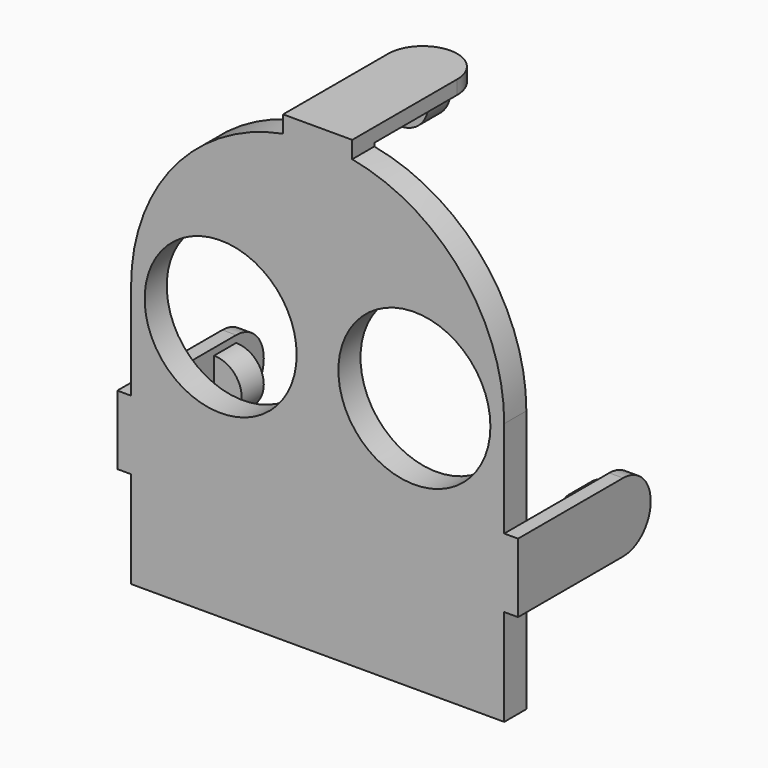
from build123d import *

# Parameters (mm, degrees)
F1_DEPTH  = 2
F4_DEPTH  = 1
F6_DEPTH  = 2
F9_DEPTH  = 1
F12_DEPTH = 1
F13_W     = 2
F13_H     = 2
F14_ANGLE = 180
F15_W     = 2
F15_H     = 2
F16_ANGLE = 180
F17_W     = 2
F17_H     = 2
F18_ANGLE = 180
F19_R     = 5.5
F20_DEPTH = 5


# Not quite as in the source:
# - a feature names something its author has since deleted; it is built from what else it names


with BuildPart() as f1:
    # F0 (on Front) → F1 (new body)
    with BuildSketch(Plane.XZ):
        with BuildLine():
            ThreePointArc((-13.5, 0), (0, -13.5), (13.5, 0))
            ThreePointArc((13.5, 0), (0, 13.5), (-13.5, 0))
        make_face()
        with BuildLine():
            Line((13.5, -19), (13.5, 0))
            ThreePointArc((13.5, 0), (0, -13.5), (-13.5, 0))
            Line((-13.5, 0), (-13.5, -19))
            Line((-13.5, -19), (13.5, -19))
        make_face()
    extrude(amount=F1_DEPTH)

    # F3 (on offset) → F4 (join)
    with BuildSketch(Plane.XY.offset(13.5)):
        with BuildLine():
            Line((-2.5, 7.5), (-2.5, -2))
            Line((-2.5, -2), (2.5, -2))
            Line((2.5, -2), (2.5, 7.5))
            ThreePointArc((2.5, 7.5), (1.767766953, 9.267766953), (0, 10))
            ThreePointArc((0, 10), (-1.767766953, 9.267766953), (-2.5, 7.5))
        make_face()
    extrude(amount=F4_DEPTH)

    # F5 (on face) → F6 (join)
    with BuildSketch(Plane.XZ.offset(2)):
        with BuildLine():
            Line((-2.5, 13.5), (-2.5, 13.2664991614))
            ThreePointArc((-2.5, 13.2664991614), (-1.2554404249, 13.4414980318), (0, 13.5))
            Line((0, 13.5), (-2.5, 13.5))
        make_face()
        with BuildLine():
            ThreePointArc((0, 13.5), (1.2554404249, 13.4414980318), (2.5, 13.2664991614))
            Line((2.5, 13.2664991614), (2.5, 13.5))
            Line((2.5, 13.5), (0, 13.5))
        make_face()
    extrude(amount=-F6_DEPTH)

    # F8 (on offset) → F9 (join)
    with BuildSketch(Plane.YZ.offset(13.5)):
        with BuildLine():
            Line((7.5, -7), (-2, -7))
            Line((-2, -7), (-2, -12))
            Line((-2, -12), (7.5, -12))
            ThreePointArc((7.5, -12), (9.267766953, -11.267766953), (10, -9.5))
            ThreePointArc((10, -9.5), (9.267766953, -7.732233047), (7.5, -7))
        make_face()
    extrude(amount=F9_DEPTH)

    # F11 (on offset) → F12 (join)
    with BuildSketch(Plane.YZ.offset(-13.5)):
        with BuildLine():
            Line((7.5, -7), (-2, -7))
            Line((-2, -7), (-2, -12))
            Line((-2, -12), (7.5, -12))
            ThreePointArc((7.5, -12), (9.267766953, -11.267766953), (10, -9.5))
            ThreePointArc((10, -9.5), (9.267766953, -7.732233047), (7.5, -7))
        make_face()
    extrude(amount=-F12_DEPTH)

    # F13 (on face) → F14 (revolve)
    with BuildSketch(Plane(origin=(0, 0, 13.5), x_dir=(1, 0, 0), z_dir=(0, 0, -1))):
        with Locations((-1, -6.5)):
            Rectangle(F13_W, F13_H)
    revolve(axis=Axis((0, 6.5, 13.5), (0, -1, 0)), revolution_arc=F14_ANGLE)

    # F15 (on face) → F16 (revolve)
    with BuildSketch(Plane(origin=(13.5, 0, 0), x_dir=(0, -1, 0), z_dir=(-1, 0, 0))):
        with Locations((-6.5, -8.5)):
            Rectangle(F15_W, F15_H)
    revolve(axis=Axis((13.5, 6.5, -9.5), (0, -1, 0)), revolution_arc=F16_ANGLE)

    # F17 (on face) → F18 (revolve)
    with BuildSketch(Plane.YZ.offset(-13.5)):
        with Locations((6.5, -8.5)):
            Rectangle(F17_W, F17_H)
    revolve(axis=Axis((-13.5, 6.5, -9.5), (0, 1, 0)), revolution_arc=F18_ANGLE)

    # F19 (on face) → F20 (cut)
    with BuildSketch(Plane.XZ.offset(2)):
        with Locations((-7.0192593016, -0.5)):
            Circle(F19_R)
        with Locations((7, -0.5)):
            Circle(F19_R)
    extrude(amount=-F20_DEPTH, mode=Mode.SUBTRACT)


solid = f1.part
